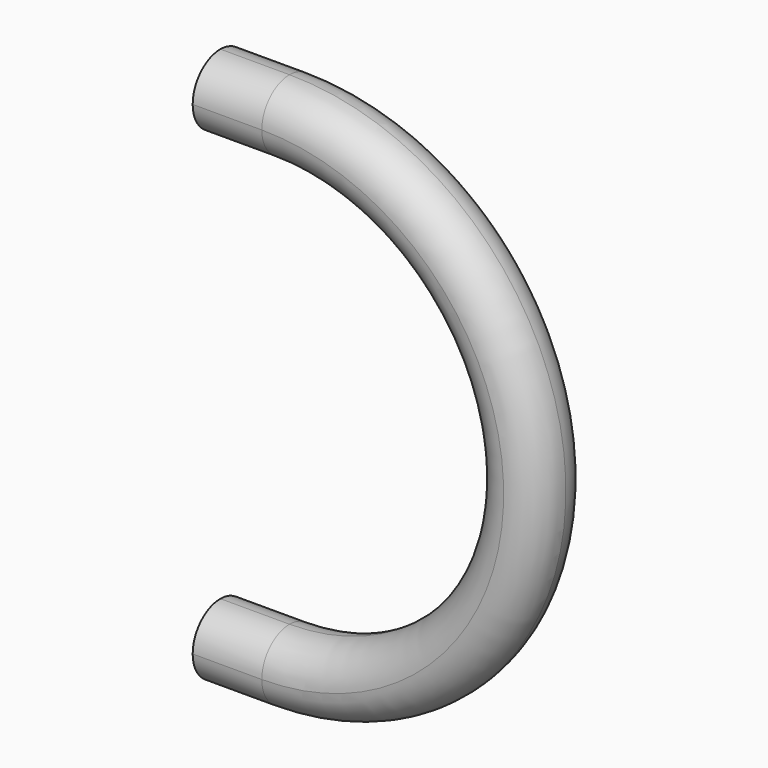
from build123d import *

# Parameters (mm, degrees)
F1_DEPTH = 6.35
F2_R     = 3.17499


# Not quite as in the source:
# - a fillet or chamfer is up to 0.001 mm smaller than in the source, because OpenCascade refuses the exact size


with BuildPart() as f1:
    # F0 (on Front) → F1 (new body)
    with BuildSketch(Plane.XZ):
        with BuildLine():
            Line((0, 6.350000307), (0, 0))
            Line((0, 0), (6.35, 0))
            ThreePointArc((6.35, 0), (31.75, 25.4), (6.35, 50.8))
            Line((6.35, 50.8), (0, 50.8))
            Line((0, 50.8), (0, 44.449999693))
            Line((0, 44.449999693), (6.35, 44.449999693))
            ThreePointArc((6.35, 44.449999693), (25.399999693, 25.4), (6.35, 6.350000307))
            Line((6.35, 6.350000307), (0, 6.350000307))
        make_face()
    extrude(amount=F1_DEPTH)

    # F2 (radius 3.175 in the source; OpenCascade refuses exactly that, so slightly less here)
    f2_edges = [f1.edges().sort_by_distance(p)[0] for p in [
        (31.75, -6.35, 25.4),
        (25.4, -6.35, 25.4),
        (31.75, 0, 25.4),
        (3.175, 0, 6.35),
    ]]
    fillet(f2_edges, radius=F2_R)


solid = f1.part
